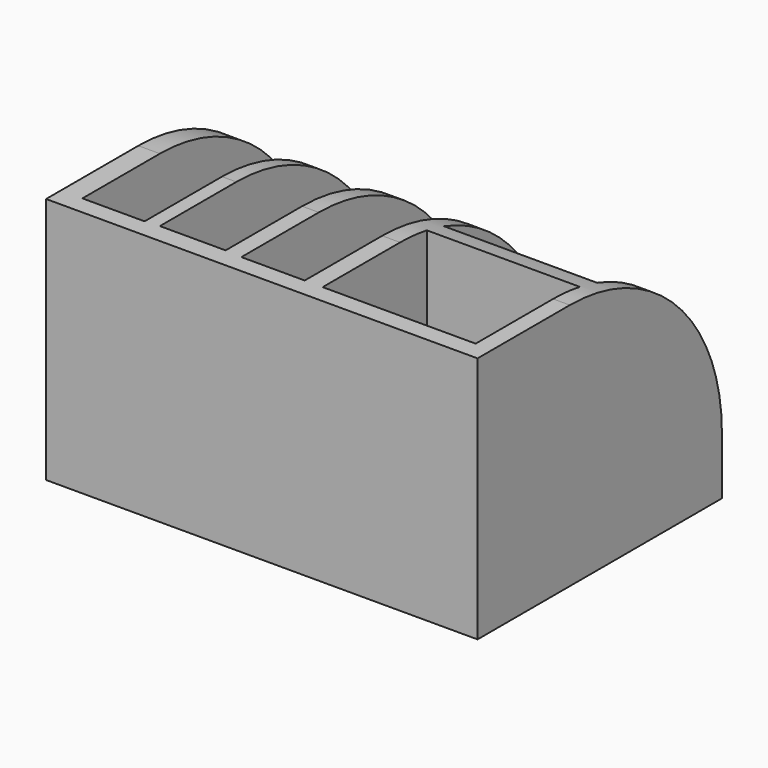
from build123d import *

# Parameters (mm, degrees)
F0_W        = 102.9718667269
F0_H        = 59.044812806
F1_DEPTH    = 72.898
F2_W        = 14.8325152695
F2_H        = 63.3234274574
F2_W_2      = 15.6882368028
F2_H_2      = 63.3234172128
F2_W_3      = 15.1177551597
F2_H_3      = 63.8939035125
F2_W_4      = 36.5108018741
F2_H_4      = 27.9535762966
F2_H_5      = 31.0912323184
F4_DEPTH    = 47.498
F5_T1_DEPTH = 329.8596573187


# Not quite as in the source:
# - a fillet or chamfer that OpenCascade refuses, or shapes differently, is made with other operations: its cross-section is extruded or revolved along the edge and cut away or added


with BuildPart() as f1:
    # F0 (on Front) → F1 (new body)
    with BuildSketch(Plane.XZ):
        with Locations((0.1426190138, -18.5406408273)):
            Rectangle(F0_W, F0_H)
    extrude(amount=-F1_DEPTH)

    # F2 (on face) → F4 (cut)
    with BuildSketch(Plane.XY.offset(10.9817655757)):
        with Locations((-38.7927275151, 36.0829436686)):
            Rectangle(F2_W, F2_H)
        with Locations((-20.1094653457, 36.3681793679)):
            Rectangle(F2_W_2, F2_H_2)
        with Locations((-0.7131015882, 36.3681816962)):
            Rectangle(F2_W_3, F2_H_3)
        with Locations((29.3797855265, 54.6235833317)):
            Rectangle(F2_W_4, F2_H_4)
        with Locations((29.3797855265, 19.9668460991)):
            Rectangle(F2_W_4, F2_H_5)
    extrude(amount=-F4_DEPTH, mode=Mode.SUBTRACT)

    # F5: fillet of radius 45.3775581184 on 1 edges, made by hand

    # F5_s2 → F5_t1 (cut)
    with BuildSketch(Plane.YZ.offset(-164.7872096456)):
        with BuildLine():
            ThreePointArc((27.5204418816, 10.9817655757), (59.6072209408, -2.3090134835), (72.898, -34.3957925427))
            Line((72.898, -34.3957925427), (72.898, 10.9817655757))
            Line((72.898, 10.9817655757), (27.5204418816, 10.9817655757))
        make_face()
    extrude(amount=F5_T1_DEPTH, mode=Mode.SUBTRACT)


solid = f1.part
